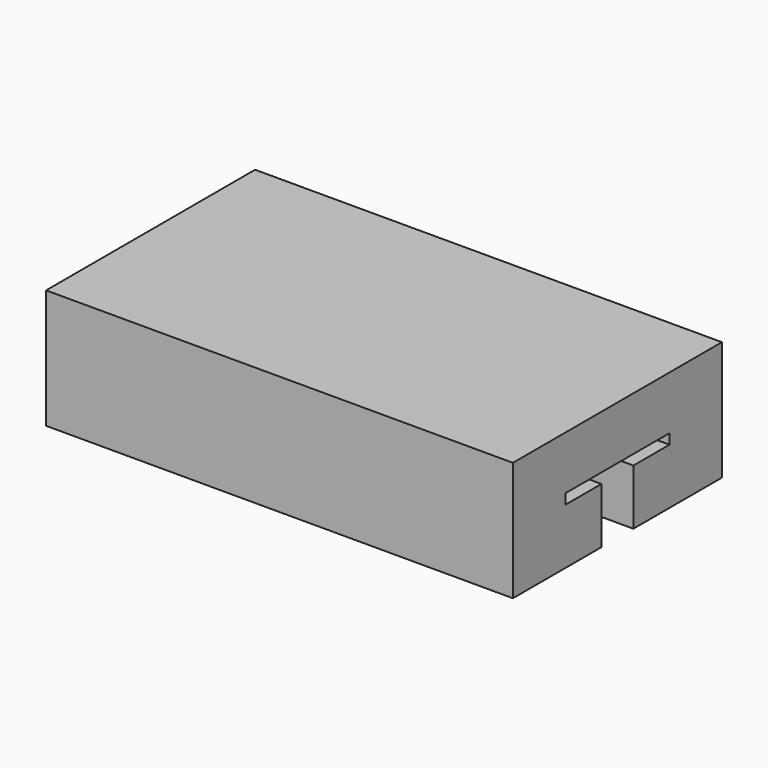
from build123d import *

# Parameters (mm, degrees)
F0_W     = 31.6056316875
F0_H     = 12
F1_DEPTH = 25
F2_W     = 8.3738705143
F2_H     = 14.6988127381
F3_DEPTH = 166
F4_W     = 7.847521259
F4_H     = 27.2596180439
F5_DEPTH = 5


# Not quite as in the source:
# - an extrude ends at something that could not be found from the text; its depth is read off the source's solid


with BuildPart() as f1:
    # F0 (on Top) → F1 (new body)
    with BuildSketch(Plane.XY):
        Polygon((48.9295756356, -27.3802791548), (48.9295756356, 27.3802791548), (-48.9295756356, 27.3802791548), (-48.9295756356, 6), (-17.3239439482, 6), (-17.3239439482, -6), (-48.9295756356, -6), (-48.9295756356, -27.3802791548), align=None)
        with Locations((-33.1267597919, 0)):
            Rectangle(F0_W, F0_H)
    extrude(amount=F1_DEPTH)

    # F2 (on face) → F3 (cut, through all)
    with BuildSketch(Plane.YZ.offset(48.9295756356)):
        with Locations((0, -7.349406369)):
            Rectangle(F2_W, F2_H)
        Polygon((13.6298090219, 11.6699673235), (13.6298090219, 18.7966637313), (-13.6298090219, 18.7966637313), (-13.6298090219, 11.6699673235), (-4.1869352572, 11.6699673235), (-4.1869352572, 0), (4.1869352572, 0), (4.1869352572, 11.6699673235), align=None)
    extrude(amount=-F3_DEPTH, mode=Mode.SUBTRACT)

    # F4 (on face) → F5 (join)
    with BuildSketch(Plane(origin=(0, 0, 18.7966637313), x_dir=(1, 0, 0), z_dir=(0, 0, -1))):
        with Locations((-45.0058150061, 0)):
            Rectangle(F4_W, F4_H)
        with Locations((45.0058150061, 0)):
            Rectangle(F4_W, F4_H)
    extrude(amount=F5_DEPTH)


solid = f1.part
